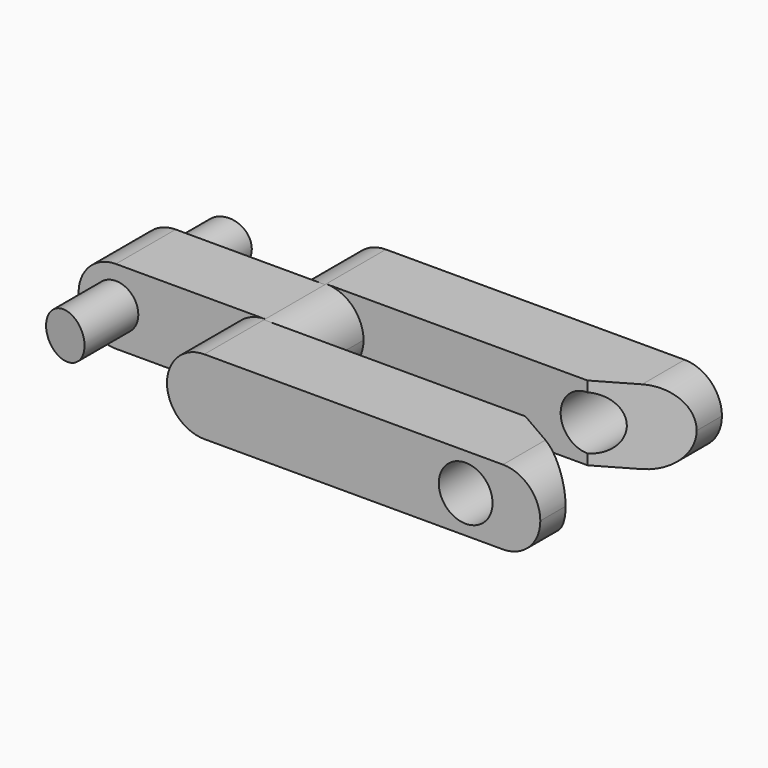
from build123d import *

# Parameters (mm, degrees)
F1_DEPTH = 1.5875
F3_DEPTH = 4.445
F4_R     = 1.58749
F5_R     = 1.143
F6_DEPTH = 12.7
F8_DEPTH = 12.7


# Not quite as in the source:
# - a fillet or chamfer is up to 0.001 mm smaller than in the source, because OpenCascade refuses the exact size


with BuildPart() as f1:
    # F0 (on Top) → F1 (new body, symmetric)
    with BuildSketch(Plane.XY):
        Polygon((12.7, 1.651), (12.7, 4.826), (-3.175, 4.826), (-3.175, 1.5875), (-9.525, 1.5875), (-9.525, -1.5875), (-3.175, -1.5875), (-3.175, -4.826), (12.7, -4.826), (12.7, -1.651), (0, -1.651), (0, 0), (0, 1.651), align=None)
    extrude(amount=F1_DEPTH, both=True)

    # F2 (on Front) → F3 (join, symmetric)
    with BuildSketch(Plane.XZ):
        with BuildLine():
            ThreePointArc((-8.89, 0), (-7.9375, -0.9525), (-6.985, 0))
            ThreePointArc((-6.985, 0), (-7.9375, 0.9525), (-8.89, 0))
        make_face()
    extrude(amount=F3_DEPTH, both=True)

    # F4 (radius 1.5875 in the source; OpenCascade refuses exactly that, so slightly less here)
    f4_edges = [f1.edges().sort_by_distance(p)[0] for p in [
        (-3.175, 3.20675, -1.5875),
        (-3.175, 3.20675, 1.5875),
        (-3.175, -3.20675, 1.5875),
        (-3.175, -3.20675, -1.5875),
        (-9.525, 0, 1.5875),
        (-9.525, 0, -1.5875),
        (12.7, 3.2385, -1.5875),
        (12.7, 3.2385, 1.5875),
        (12.7, -3.2385, 1.5875),
        (12.7, -3.2385, -1.5875),
        (0, 0, 1.5875),
        (0, 0, -1.5875),
    ]]
    fillet(f4_edges, radius=F4_R)

    # F5 (on Front) → F6 (cut, symmetric)
    with BuildSketch(Plane.XZ):
        with Locations((9.525, 0)):
            Circle(F5_R)
    extrude(amount=F6_DEPTH, both=True, mode=Mode.SUBTRACT)

    # F7 (on Top) → F8 (cut, symmetric)
    with BuildSketch(Plane.XY):
        Polygon((9.525, 1.651), (9.525, -1.651), (15.875, -5.3171742094), (15.875, 5.3171742094), align=None)
        Polygon((-9.525, 4.445), (-9.525, 3.997129469), (-6.985, 4.445), align=None)
        Polygon((-9.525, -4.445), (-6.985, -4.445), (-9.525, -3.997129469), align=None)
    extrude(amount=F8_DEPTH, both=True, mode=Mode.SUBTRACT)


solid = f1.part
